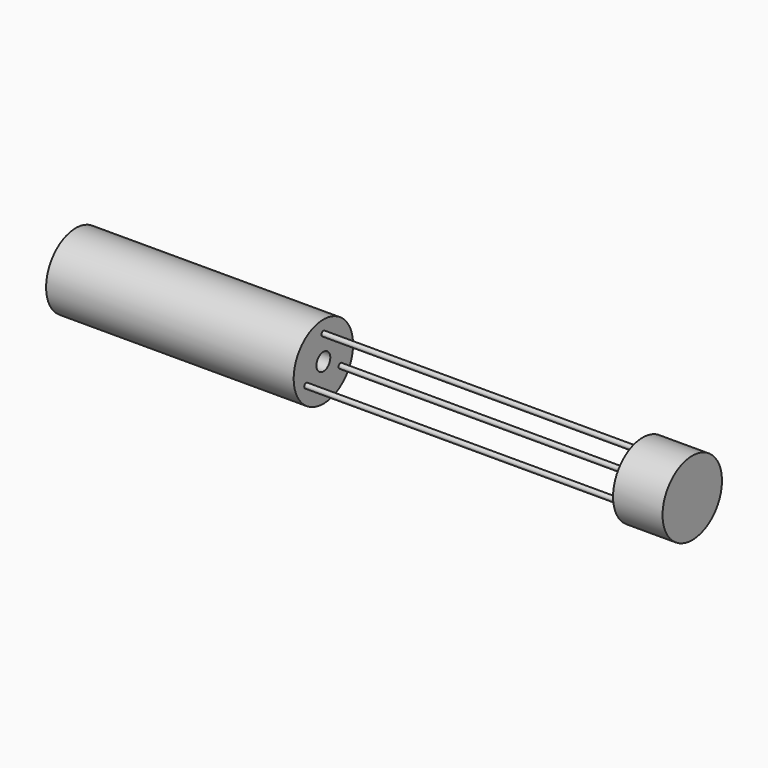
from build123d import *

# Parameters (mm, degrees)
F1_W     = 100
F1_H     = 75
F3_R     = 5
F4_DEPTH = 645


# Not quite as in the source:
# - a feature names something its author has since deleted; it is built from what else it names


with BuildPart() as f2:
    # F0 (on Top) → F2 (revolve)
    with BuildSketch(Plane.XY):
        Polygon((-200, 0), (-500, 0), (-500, -75), (0, -75), (0, -17.5), (-200, -17.5), align=None)
    revolve(axis=Axis((-350, 0, 0), (-1, 0, 0)))


with BuildPart() as f2b:
    # F1 (on Top) → F2, piece 2 (revolve)
    with BuildSketch(Plane.XY):
        with Locations((695, -37.5)):
            Rectangle(F1_W, F1_H)
    revolve(axis=Axis((-350, 0, 0), (-1, 0, 0)))


with BuildPart() as f4:
    # F3 (on Right) → F4 (new body, through all)
    with BuildSketch(Plane.YZ):
        with Locations((0, 50)):
            Circle(F3_R)
    extrude(amount=F4_DEPTH)


with BuildPart() as f4b:
    # F3 (on Right) → F4, piece 2 (new body, through all)
    with BuildSketch(Plane.YZ):
        with Locations((-43.3012701892, -25)):
            Circle(F3_R)
    extrude(amount=F4_DEPTH)


with BuildPart() as f4c:
    # F3 (on Right) → F4, piece 3 (new body, through all)
    with BuildSketch(Plane.YZ):
        with Locations((43.3012701892, -25)):
            Circle(F3_R)
    extrude(amount=F4_DEPTH)


solid = Compound([f2.part, f2b.part, f4.part, f4b.part, f4c.part])
